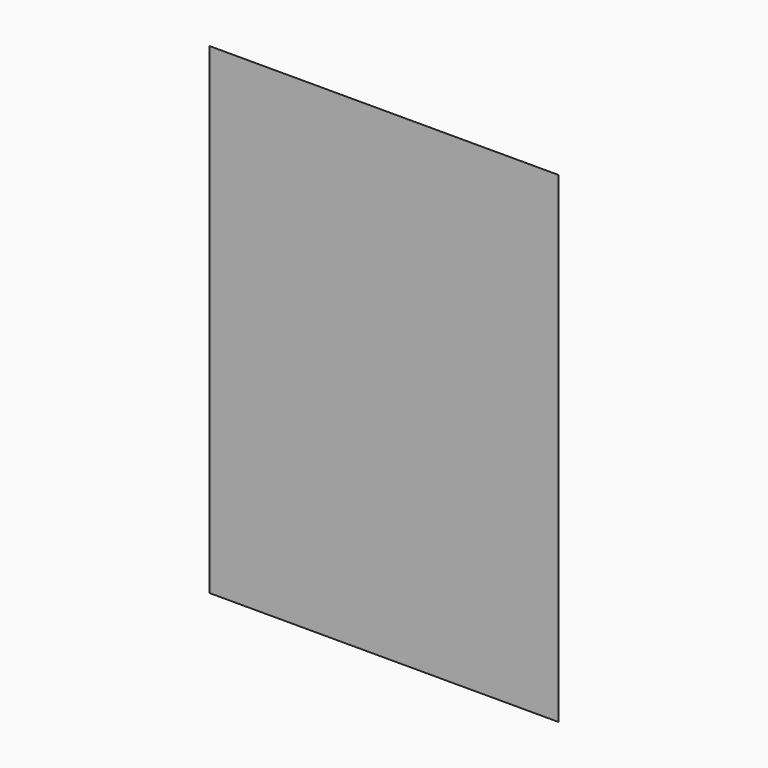
from build123d import *

# Parameters (mm, degrees)
F0_W     = 24.0014512092
F0_H     = 33.1514887512
F1_DEPTH = 5
F2_SIZE  = 4.99999


# Not quite as in the source:
# - a fillet or chamfer is up to 0.001 mm smaller than in the source, because OpenCascade refuses the exact size


with BuildPart() as f1:
    # F0 (on Front) → F1 (new body)
    with BuildSketch(Plane.XZ):
        Rectangle(F0_W, F0_H)
    extrude(amount=F1_DEPTH)

    # F2 (size 5 in the source; OpenCascade refuses exactly that, so slightly less here)
    f2_edges = [f1.edges().sort_by_distance(p)[0] for p in [
        (-12.000726, 0, 0),
        (0, 0, 16.575744),
        (0, 0, -16.575744),
        (12.000726, 0, 0),
    ]]
    chamfer(f2_edges, length=F2_SIZE)


solid = f1.part
